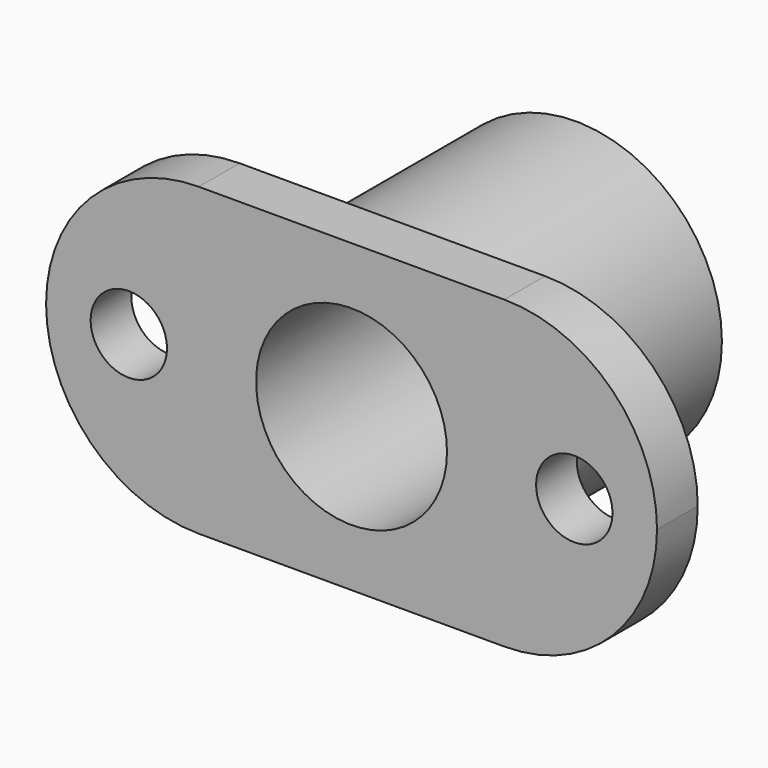
from build123d import *

# Parameters (mm, degrees)
F0_R     = 5.75
F0_R_2   = 3.75
F1_DEPTH = 11
F2_W     = 24
F2_H     = 12
F2_R     = 5.75
F3_DEPTH = 2
F4_D     = 3
F5_R     = 5.99999


# Not quite as in the source:
# - a fillet or chamfer is up to 0.001 mm smaller than in the source, because OpenCascade refuses the exact size


with BuildPart() as f1:
    # F0 (on Front) → F1 (new body)
    with BuildSketch(Plane.XZ):
        Circle(F0_R)
        Circle(F0_R_2, mode=Mode.SUBTRACT)
    extrude(amount=F1_DEPTH)

    # F2 (on face) → F3 (join)
    with BuildSketch(Plane.XZ.offset(11)):
        Rectangle(F2_W, F2_H)
        Circle(F2_R, mode=Mode.SUBTRACT)
    extrude(amount=-F3_DEPTH)

    # F4 (through all)
    with Locations(Plane.XZ.offset(11)):
        with Locations((-8.75, 0), (8.75, 0)):
            Hole(F4_D / 2)

    # F5 (radius 6 in the source; OpenCascade refuses exactly that, so slightly less here)
    f5_edges = [f1.edges().sort_by_distance(p)[0] for p in [
        (12, -10, 6),
        (12, -10, -6),
        (-12, -10, 6),
        (-12, -10, -6),
    ]]
    fillet(f5_edges, radius=F5_R)


solid = f1.part
